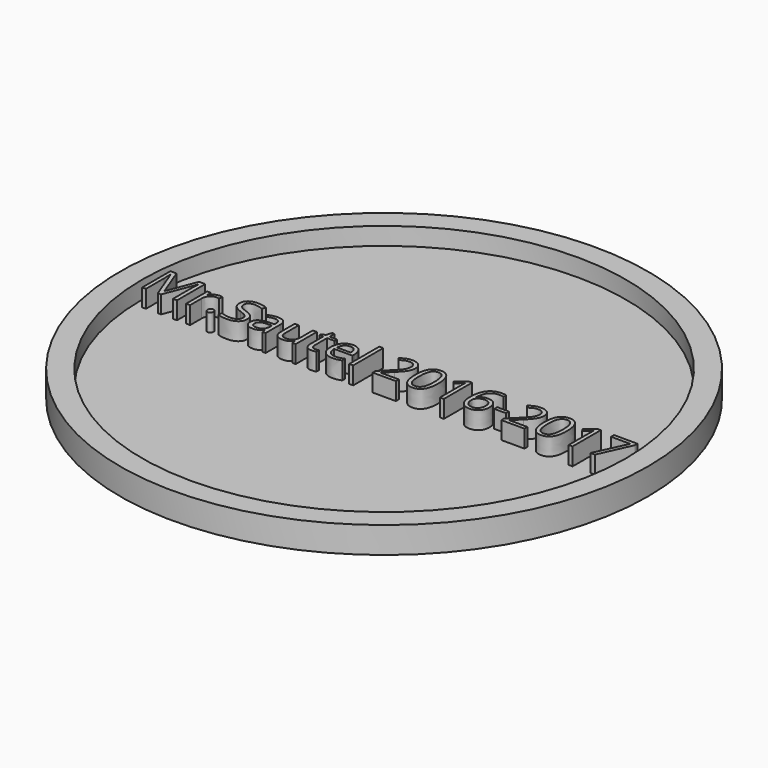
from build123d import *

# Parameters (mm, degrees)
F0_R         = 38.1
F1_DEPTH     = 3.81
F2_R         = 34.925
F3_DEPTH     = 2.54
F4_TEXT_SIZE = 7.1197625189
F5_DEPTH     = 2.54


# Not quite as in the source:
# - Text() gives the source's letters only with a copy of the font that has no kerning and outlines rounded to 1/6400 em; it was checked with that copy


with BuildPart() as f1:
    # F0 (on Top) → F1 (new body)
    with BuildSketch(Plane.XY):
        Circle(F0_R)
    extrude(amount=F1_DEPTH)

    # F2 (on face) → F3 (cut)
    with BuildSketch(Plane.XY.offset(3.81)):
        Circle(F2_R)
    extrude(amount=-F3_DEPTH, mode=Mode.SUBTRACT)

    # F4 (on face) → F5 (join)
    with BuildSketch(Plane.XY.offset(1.27)):
        with Locations((-34.4231462737, -1.4891373867)):
            Text('Mr.Sautel 2016-2017', F4_TEXT_SIZE, font='Open Sans', text_align=(TextAlign.LEFT, TextAlign.BOTTOM))
    extrude(amount=F5_DEPTH)


solid = f1.part
